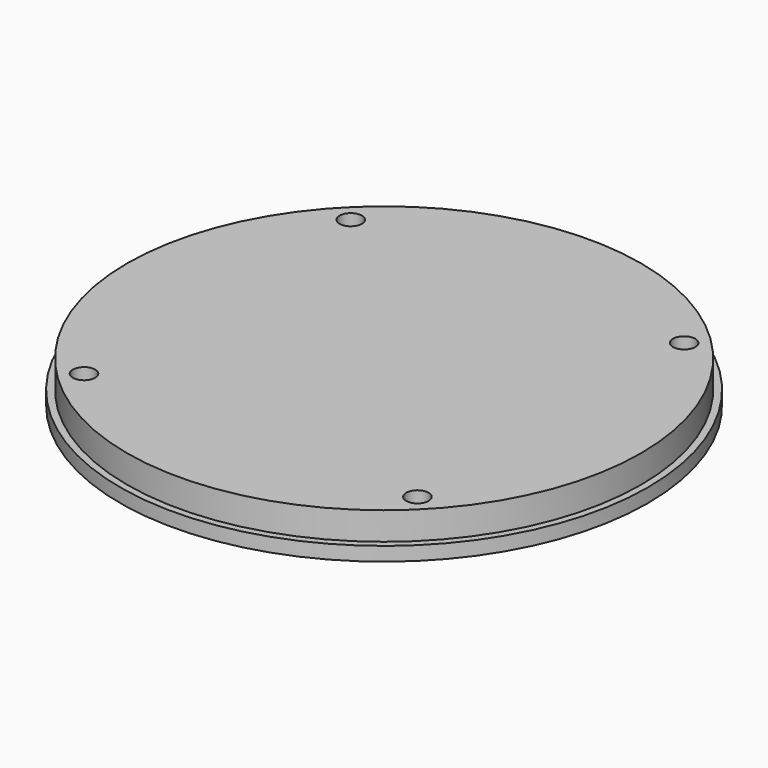
from build123d import *

# Parameters (mm, degrees)
F0_R     = 60.325
F0_R_2   = 58.7375
F1_DEPTH = 3.175
F2_DEPTH = 9.525
F3_D     = 5.1054
F3_DEPTH = 76.2
F3_TIP   = 1.5338169022


# Not quite as in the source:
# - a feature names something its author has since deleted; it is built from what else it names


with BuildPart() as f1:
    # F0 (on Top) → F1 (new body)
    with BuildSketch(Plane.XY):
        Circle(F0_R)
        Circle(F0_R_2, mode=Mode.SUBTRACT)
        Circle(F0_R_2)
    extrude(amount=F1_DEPTH)

    # F0 (on Top) → F2 (join)
    with BuildSketch(Plane.XY):
        Circle(F0_R_2)
    extrude(amount=F2_DEPTH)

    # F3
    with Locations(Plane(origin=(0, 0, 0), x_dir=(1, 0, 0), z_dir=(0, 0, -1))):
        with Locations((38.1, -38.1), (-38.1, -38.1), (-38.1, 38.1), (38.1, 38.1)):
            Hole(F3_D / 2, depth=F3_DEPTH)
            with Locations((0, 0, -(F3_DEPTH + F3_TIP / 2))):  # 118° drill point
                Cone(0, F3_D / 2, F3_TIP, mode=Mode.SUBTRACT)


solid = f1.part
